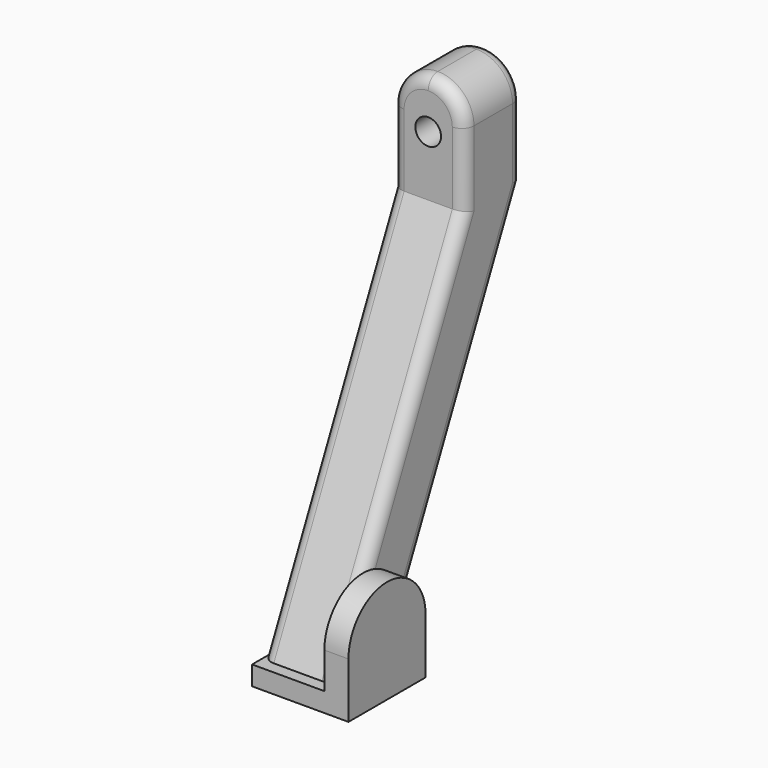
from build123d import *

# Parameters (mm, degrees)
F1_W      = 6
F1_H      = 6
F2_DEPTH  = 1.2
F5_DEPTH  = 2.25
F6_R      = 0.8
F7_DEPTH  = 15.3931915649
F8_R      = 2.24999
F9_R      = 0.75
F11_DEPTH = 1.5


# Not quite as in the source:
# - a fillet or chamfer is up to 0.001 mm smaller than in the source, because OpenCascade refuses the exact size


with BuildPart() as f2:
    # F1 (on Top) → F2 (new body)
    with BuildSketch(Plane.XY):
        with Locations((4.5, 3)):
            Rectangle(F1_W, F1_H)
    extrude(amount=F2_DEPTH)

    # F4 (on offset) → F5 (join, symmetric)
    with BuildSketch(Plane.YZ.offset(3.75)):
        Polygon((0.75, 1.2), (5.25, 1.2), (15.3921915649, 22.95), (15.3921915649, 29.7), (10.8921915649, 29.7), (10.8921915649, 22.95), align=None)
    extrude(amount=F5_DEPTH, both=True)

    # F6 (on face) → F7 (cut, through all)
    with BuildSketch(Plane(origin=(0, 15.3921915649, 0), x_dir=(-1, 0, 0), z_dir=(0, 1, 0))):
        with Locations((-3.75, 26.7)):
            Circle(F6_R)
    extrude(amount=-F7_DEPTH, mode=Mode.SUBTRACT)

    # F8 (radius 2.25 in the source; OpenCascade refuses exactly that, so slightly less here)
    f8_edges = [f2.edges().sort_by_distance(p)[0] for p in [
        (1.5, 13.142192, 29.7),
        (6, 13.142192, 29.7),
    ]]
    fillet(f8_edges, radius=F8_R)

    # F9
    f9_edges = [f2.edges().sort_by_distance(p)[0] for p in [
        (1.5, 10.321096, 12.075),
        (1.5, 15.392192, 25.200005),
        (5.340993, 15.392192, 29.040993),
        (6, 10.321096, 12.075),
        (1.5, 5.821096, 12.075),
        (1.5, 10.892192, 25.200005),
        (6, 5.821096, 12.075),
    ]]
    fillet(f9_edges, radius=F9_R)

    # F10 (on face) → F11 (join)
    with BuildSketch(Plane.YZ.offset(7.5)):
        with BuildLine():
            Line((0, 3.45), (0, 1.2))
            Line((0, 1.2), (6, 1.2))
            Line((6, 1.2), (6, 3.45))
            ThreePointArc((6, 3.45), (3, 6.45), (0, 3.45))
        make_face()
    extrude(amount=-F11_DEPTH)


solid = f2.part
